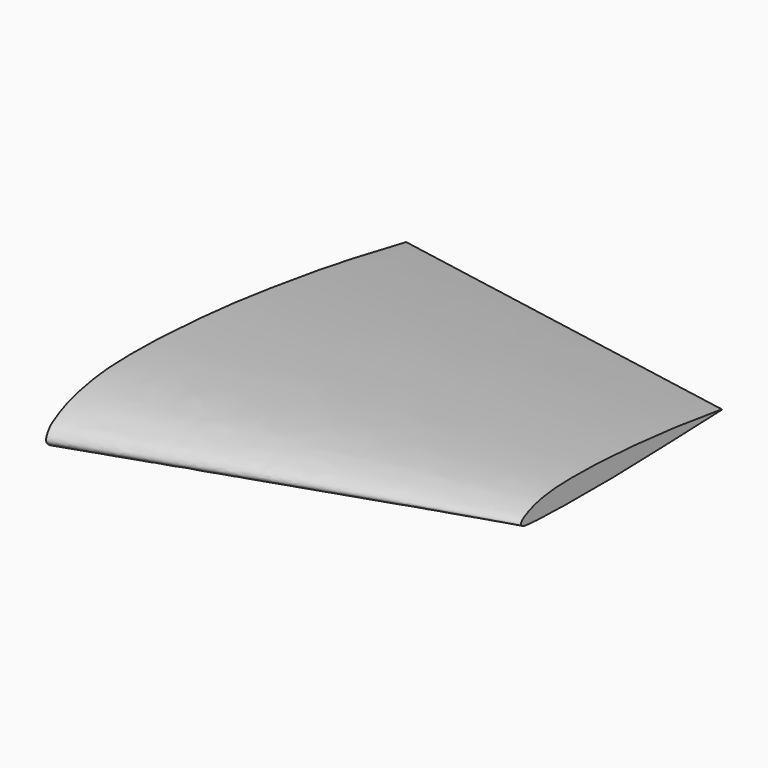
from build123d import *


with BuildPart() as f9:
    # F7 (on face) → F9 section 0
    with BuildSketch(Plane(origin=(2789.5608593403, 0, 293.194660848), x_dir=(0, -1, 0), z_dir=(-0.9945218954, 0, -0.1045284633))):
        with BuildLine():
            add(Edge.make_bspline(
                [(-1674.9361309886, -107.9427576127), (-1637.4672962285, -100.8277234072), (-1562.5593562878, -86.6033004074), (-1453.1073844063, -66.9731191492), (-1230.4334752707, -29.1693149363), (-1017.9593413467, 0.8000957791), (-796.8935594426, 29.1031628485), (-575.7328245472, 53.1020212502), (-363.093637858, 68.513103179), (-139.5744105016, 78.8856014184), (-30.3074510706, 79.6465607408), (84.5131751526, 78.2709351665), (190.3544656586, 71.423301684), (302.4963815785, 52.2941834439), (357.9407868905, 37.6440452339), (413.4967752298, 20.788669365), (470.5566325035, -7.2068104015), (496.7947946717, -21.5032951955), (541.6713617639, -75.1004607385), (497.3399259613, -104.2604378308), (471.8847837935, -113.347137273), (415.431934254, -125.6323119565), (360.5483778662, -130.8146198497), (305.4227754367, -138.2043317621), (193.7026937829, -146.4660001933), (88.3842122177, -153.0277142593), (-26.3275714215, -156.2553564371), (-135.4466799784, -162.4176581974), (-359.1185599884, -163.3825437775), (-572.0093390245, -160.5487067399), (-793.6953612013, -153.6277291235), (-1015.393547331, -145.6033386135), (-1228.4420680323, -136.9011778967), (-1452.0477715375, -125.6682627238), (-1561.9660286955, -120.1074109507), (-1637.2154322096, -115.5506876895), (-1674.845681882, -113.2719901052)],
                knots=[0, 0, 0, 0, 0.0281929138, 0.056363458, 0.096165249, 0.1359079799, 0.1756106035, 0.2152726592, 0.2548893878, 0.2944818259, 0.3224715986, 0.3504708764, 0.3785199609, 0.4067405213, 0.4268781172, 0.4472523654, 0.4681178147, 0.4835524873, 0.5034392763, 0.5201851584, 0.5346345515, 0.5546114688, 0.5744586317, 0.5942967281, 0.6223147737, 0.6503164573, 0.6783103546, 0.7063037045, 0.7458887493, 0.7854827471, 0.8250880218, 0.8647001136, 0.9043185332, 0.9439455018, 0.9719686182, 1, 1, 1, 1], degree=3))
            ThreePointArc((-1674.9361309886, -107.9427576127), (-1677.1355304311, -110.6454701955), (-1674.845681882, -113.2719901052))
        make_face()
    # F8 (on face) → F9 section 1
    with BuildSketch(Plane(origin=(4896.3162616126, 0, 514.6235762957), x_dir=(0, -1, 0), z_dir=(-0.9945218954, 0, -0.1045284633))):
        with BuildLine():
            add(Edge.make_bspline(
                [(-978.9196847444, -83.5931978723), (-961.8392705884, -81.1452512028), (-915.2029971193, -74.461390421), (-728.4553589167, -50.9664895158), (-613.2379326201, -40.0811166739), (-486.2794197167, -28.310077655), (-363.2758321924, -19.7582643789), (-244.0939587157, -13.7093076956), (-119.127847265, -10.0644584827), (-58.0372038583, -11.0722216396), (6.1090975486, -11.9341399215), (65.1560565837, -15.8628313342), (127.6867107185, -24.9237361603), (158.6577574839, -31.9203252995), (189.2900858859, -41.2147021607), (221.16966069, -54.1811221482), (234.8845654493, -60.3515223716), (260.4501880091, -82.9861289582), (234.6251999677, -93.5167751698), (221.0349827114, -96.0251532461), (189.2317245017, -98.9239862156), (158.6674554628, -100.2848478199), (127.7195961076, -101.3919592376), (65.2310931887, -103.0513145144), (6.3007060663, -104.4497677698), (-57.8199420825, -105.5069924655), (-118.8883529339, -105.2827917375), (-243.901016129, -106.2604764199), (-362.8704366618, -104.1789005264), (-486.7304648596, -100.9813682749), (-610.5773175591, -97.7938646788), (-729.582799946, -94.1207736114), (-854.4794379321, -89.8440194087), (-915.8779188252, -88.2219748146), (-957.9014802316, -86.4961639626), (-978.914876113, -85.6331922049)],
                knots=[0, 0, 0, 0, 0.0288367912, 0.0787358238, 0.119429446, 0.1600982846, 0.2007396518, 0.2413568685, 0.2819574759, 0.3106625252, 0.3393691292, 0.3681132033, 0.3969664519, 0.4175114411, 0.4382905977, 0.4593416476, 0.4746597444, 0.4928401316, 0.5086738028, 0.5231884904, 0.5435272942, 0.5638370231, 0.5841396779, 0.6128486717, 0.6415562856, 0.6702596041, 0.6989641603, 0.739558533, 0.780155668, 0.820757339, 0.8613585564, 0.9019639746, 0.9425708522, 0.9712832188, 1, 1, 1, 1], degree=3))
            ThreePointArc((-978.9196847444, -83.5931978723), (-979.8036227246, -84.6152843059), (-978.914876113, -85.6331922049))
        make_face()
    loft()


solid = f9.part
